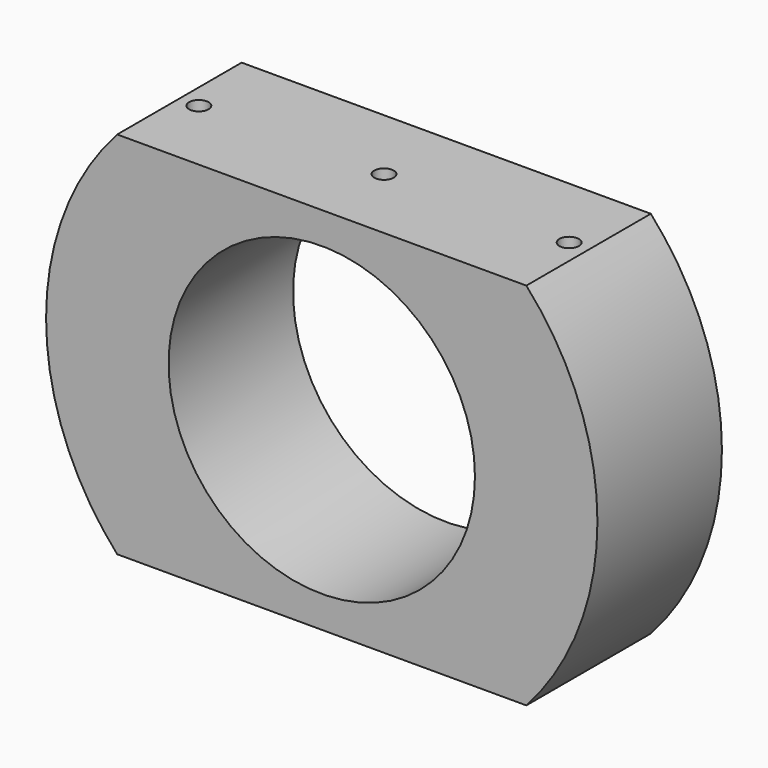
from build123d import *

# Parameters (mm, degrees)
F0_R     = 45
F1_DEPTH = 12.7
F3_DEPTH = 25.401
F4_R     = 25.00625
F5_DEPTH = 25.401
F6_R     = 1.5875
F7_DEPTH = 50.8


# Not quite as in the source:
# - a feature names something its author has since deleted; it is built from what else it names


with BuildPart() as f1:
    # F0 (on Front) → F1 (new body, symmetric)
    with BuildSketch(Plane.XZ):
        Circle(F0_R)
    extrude(amount=F1_DEPTH, both=True)

    # F2 (on face) → F3 (cut, through all)
    with BuildSketch(Plane.XZ.offset(12.7)):
        with BuildLine():
            Line((-33.3949635986, 30.1625), (33.3949635986, 30.1625))
            ThreePointArc((33.3949635986, 30.1625), (0, 45), (-33.3949635986, 30.1625))
        make_face()
        with BuildLine():
            ThreePointArc((-33.3949635986, -30.1625), (0, -45), (33.3949635986, -30.1625))
            Line((33.3949635986, -30.1625), (-33.3949635986, -30.1625))
        make_face()
    extrude(amount=-F3_DEPTH, mode=Mode.SUBTRACT)

    # F4 (on face) → F5 (cut, through all)
    with BuildSketch(Plane.XZ.offset(12.7)):
        Circle(F4_R)
    extrude(amount=-F5_DEPTH, mode=Mode.SUBTRACT)

    # F6 (on face) → F7 (cut)
    with BuildSketch(Plane.XY.offset(30.1625)):
        with Locations((30.2199635986, 0)):
            Circle(F6_R)
        Circle(F6_R)
        with Locations((-30.2199635986, 0)):
            Circle(F6_R)
    extrude(amount=-F7_DEPTH, mode=Mode.SUBTRACT)


solid = f1.part
